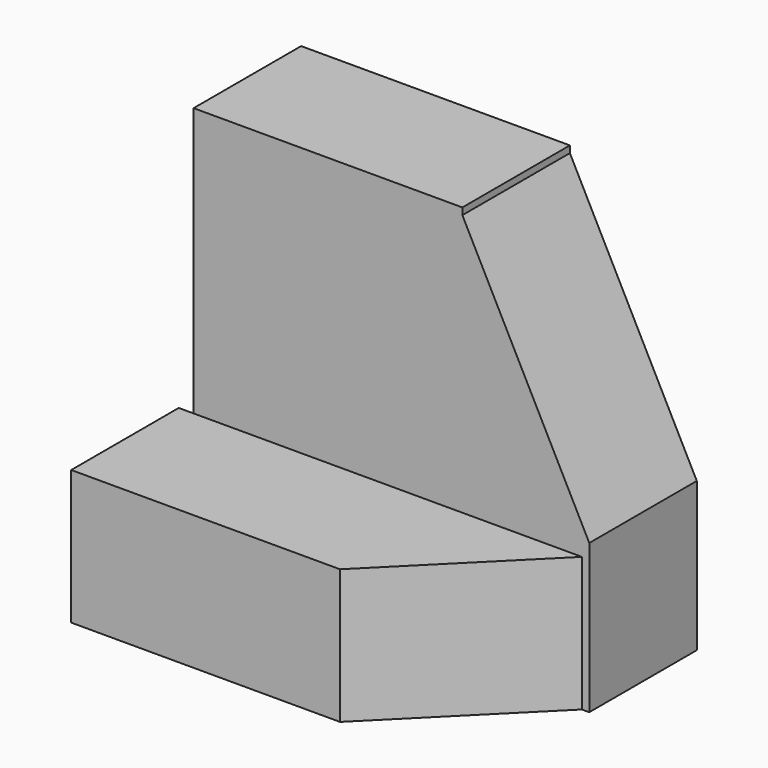
from build123d import *

# Parameters (mm, degrees)
F1_DEPTH = 12.7
F2_W     = 25.4
F2_H     = 12.7
F3_DEPTH = 38.1
F5_DEPTH = 12.7


# Not quite as in the source:
# - a feature names something its author has since deleted; it is built from what else it names


with BuildPart() as f1:
    # F0 (on Top) → F1 (new body)
    with BuildSketch(Plane.XY):
        Polygon((-9.6761901296, 0), (-47.7761901296, 0), (-47.7761901296, -12.7), (-22.3761901296, -12.7), align=None)
    extrude(amount=F1_DEPTH)

    # F2 (on Top) → F3 (join)
    with BuildSketch(Plane.XY):
        with Locations((-33.6697670078, 6.35)):
            Rectangle(F2_W, F2_H)
    extrude(amount=F3_DEPTH)

    # F4 (on Front) → F5 (join)
    with BuildSketch(Plane.XZ):
        Polygon((-21.0471171886, 37.6062467694), (-21.3566347957, 0), (-8.9759770781, 0), (-8.9759770781, 14.0829980373), align=None)
    extrude(amount=-F5_DEPTH)


solid = f1.part
